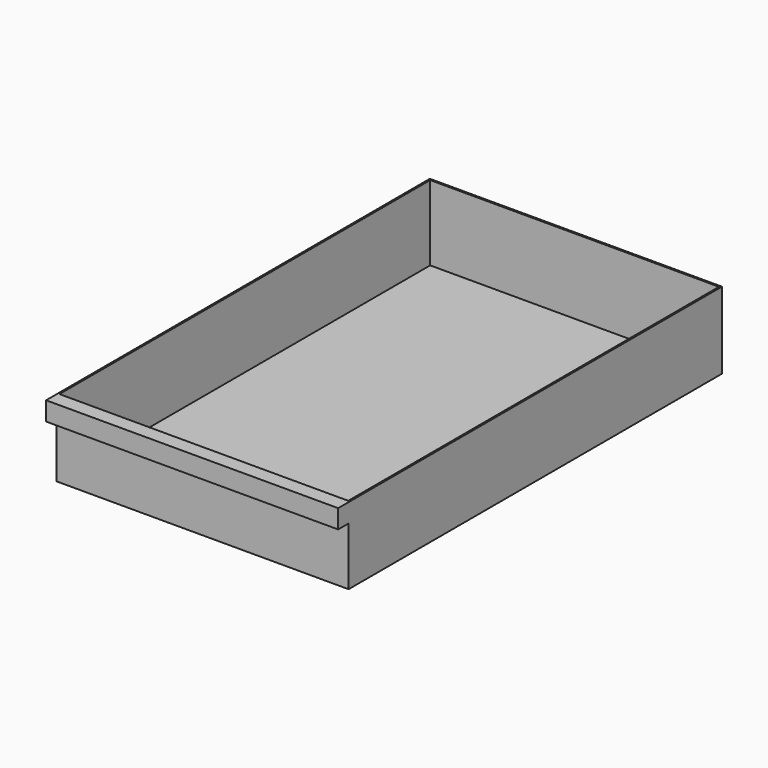
from build123d import *

# Parameters (mm, degrees)
F0_W     = 568.325
F0_H     = 149.225
F1_DEPTH = 908.05
F2_T     = -3.175
F3_W     = 568.325
F3_H     = 36.4719758213
F4_DEPTH = 25.4
F5_T     = -3.175


# Not quite as in the source:
# - a shell that OpenCascade refuses in one call is made with other operations: the cavity is built on its own and cut out


with BuildPart() as f1:
    # F0 (on Front) → F1 (new body)
    with BuildSketch(Plane.XZ):
        Rectangle(F0_W, F0_H)
    extrude(amount=F1_DEPTH)

    # F2
    f2_openings = [f1.faces().sort_by_distance(p)[0] for p in [
        (0, -454.025, 74.6125),
    ]]
    offset(amount=F2_T, openings=f2_openings)

    # F3 (on face) → F4 (join)
    with BuildSketch(Plane.XZ.offset(908.05)):
        with Locations((0, 56.3765120894)):
            Rectangle(F3_W, F3_H)
    extrude(amount=F4_DEPTH)

    # F5: a shell. OpenCascade refuses it in one call, so the cavity is built on its own and cut out:
    # the body offset inwards by the wall thickness, plus a prism from it out through each open face.
    f5_core = offset(f1.part, amount=F5_T, kind=Kind.INTERSECTION, mode=Mode.PRIVATE)
    f5_exits = [f5_core.faces().sort_by_distance(p)[0] for p in [
        (0, -919.1625, 41.315524),
    ]]
    add(f5_core, mode=Mode.SUBTRACT)
    extrude(f5_exits, amount=-F5_T, mode=Mode.SUBTRACT)


solid = f1.part
